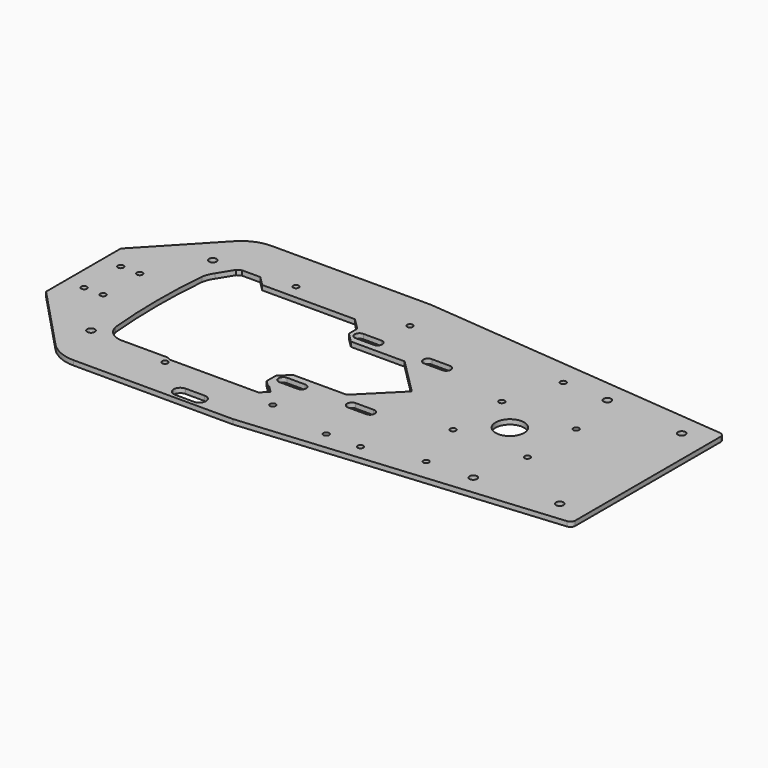
from build123d import *

# Parameters (mm, degrees)
F0_R     = 2
F0_R_2   = 1.5
F0_R_3   = 7.5
F1_DEPTH = 2.5


# Not quite as in the source:
# - ends of sketch curves that miss each other by under 0.0002 mm in the source are joined


with BuildPart() as f1:
    # F0 (on Top) → F1 (new body)
    with BuildSketch(Plane.XY):
        with BuildLine():
            Line((-115.919333, 58.73247), (-148.25, 24.5))
            Line((-148.25, 24.5), (-148.25, -24.5))
            Line((-148.25, -24.5), (-115.919333, -58.732471))
            ThreePointArc((-115.919333, -58.732471), (-109.2958427864, -63.3664016249), (-101.37907, -65))
            Line((-101.37907, -65), (-17.75, -65))
            Line((-17.75, -65), (145.974987, -50.205574))
            ThreePointArc((145.974987, -50.205574), (147.5955984677, -49.4020650272), (148.25, -47.715718))
            Line((148.25, -47.715718), (148.25, -36.5))
            Line((148.25, -36.5), (148.25, 47.715717))
            ThreePointArc((148.25, 47.715717), (147.5955984677, 49.4020640272), (145.9749869631, 50.2055725915))
            Line((145.9749869631, 50.2055725915), (-17.75, 65))
            Line((-17.75, 65), (-101.37907, 65))
            ThreePointArc((-101.37907, 65), (-109.2958431202, 63.366401481), (-115.919333, 58.73247))
        make_face()
        with Locations((-112.25, -40)):
            Circle(F0_R, mode=Mode.SUBTRACT)
        with BuildLine():
            ThreePointArc((-49.75, -63), (-52.2248737342, -61.9748737342), (-53.25, -59.5))
            ThreePointArc((-53.25, -59.5), (-52.2248737342, -57.0251262658), (-49.75, -56))
            Line((-49.75, -56), (-39.75, -56))
            ThreePointArc((-39.75, -56), (-37.2751262658, -57.0251262658), (-36.25, -59.5))
            ThreePointArc((-36.25, -59.5), (-37.2751262658, -61.9748737342), (-39.75, -63))
            Line((-39.75, -63), (-49.75, -63))
        make_face(mode=Mode.SUBTRACT)
        with Locations((-71, -43)):
            Circle(F0_R_2, mode=Mode.SUBTRACT)
        with Locations((-12.75, -45)):
            Circle(F0_R_2, mode=Mode.SUBTRACT)
        with Locations((-138.25, -12)):
            Circle(F0_R_2, mode=Mode.SUBTRACT)
        with Locations((-128.25, -12)):
            Circle(F0_R_2, mode=Mode.SUBTRACT)
        with BuildLine():
            ThreePointArc((-23.25, -27.5), (-25.017766953, -26.767766953), (-25.75, -25))
            ThreePointArc((-25.75, -25), (-25.017766953, -23.232233047), (-23.25, -22.5))
            Line((-23.25, -22.5), (-13.75, -22.5))
            ThreePointArc((-13.75, -22.5), (-11.982233047, -23.232233047), (-11.25, -25))
            ThreePointArc((-11.25, -25), (-11.982233047, -26.767766953), (-13.75, -27.5))
            Line((-13.75, -27.5), (-23.25, -27.5))
        make_face(mode=Mode.SUBTRACT)
        with Locations((20.5, -51.5)):
            Circle(F0_R_2, mode=Mode.SUBTRACT)
        with Locations((38.5, -51.5)):
            Circle(F0_R_2, mode=Mode.SUBTRACT)
        with Locations((67.75, -45)):
            Circle(F0_R_2, mode=Mode.SUBTRACT)
        with Locations((91.75, -44)):
            Circle(F0_R, mode=Mode.SUBTRACT)
        with Locations((134, -40)):
            Circle(F0_R, mode=Mode.SUBTRACT)
        with BuildLine():
            ThreePointArc((12.75, -27.5), (10.982233047, -26.767766953), (10.25, -25))
            ThreePointArc((10.25, -25), (10.982233047, -23.232233047), (12.75, -22.5))
            Line((12.75, -22.5), (22.25, -22.5))
            ThreePointArc((22.25, -22.5), (24.017766953, -23.232233047), (24.75, -25))
            ThreePointArc((24.75, -25), (24.017766953, -26.767766953), (22.25, -27.5))
            Line((22.25, -27.5), (12.75, -27.5))
        make_face(mode=Mode.SUBTRACT)
        with Locations((58.75, -16)):
            Circle(F0_R_2, mode=Mode.SUBTRACT)
        with Locations((97.75, -16)):
            Circle(F0_R_2, mode=Mode.SUBTRACT)
        with Locations((-138.25, 12)):
            Circle(F0_R_2, mode=Mode.SUBTRACT)
        with Locations((-128.25, 12)):
            Circle(F0_R_2, mode=Mode.SUBTRACT)
        with BuildLine():
            ThreePointArc((-106.6046121633, 25.7917838577), (-105.7465725985, 28.7775878211), (-104.2499995126, 31.4999996564))
            Line((-104.2499995126, 31.4999996564), (-99.481118, 39.303625))
            Line((-99.481118, 39.303625), (-97.347914, 40.5))
            Line((-97.347914, 40.5), (-87.75, 40.5))
            Line((-87.75, 40.5), (-85.25, 38))
            Line((-85.25, 38), (-82.75, 35.5))
            Line((-82.75, 35.5), (-34, 35.5))
            Line((-34, 35.5), (-28, 29.5))
            Line((-28, 29.5), (-28, 24))
            Line((-28, 24), (-23, 19))
            Line((-23, 19), (5.25, 19))
            Line((5.25, 19), (24, 0.25))
            Line((24, 0.25), (24, -0.25))
            Line((24, -0.25), (5.25, -19))
            Line((5.25, -19), (-23, -19))
            Line((-23, -19), (-28, -24))
            Line((-28, -24), (-28, -30))
            Line((-28, -30), (-25, -33))
            Line((-25, -33), (-24.25, -33))
            Line((-24.25, -33), (-20.75, -36.5))
            Line((-20.75, -36.5), (-24.25, -40))
            Line((-24.25, -40), (-70.75, -40))
            Line((-70.75, -40), (-73, -39))
            Line((-73, -39), (-96.75, -39))
            ThreePointArc((-96.75, -39), (-102.9744154707, -36.7847551324), (-106.3997748707, -31.1351909734))
            ThreePointArc((-106.3997748707, -31.1351909734), (-107.7934268918, -2.6763496917), (-106.6046121633, 25.7917838577))
        make_face(mode=Mode.SUBTRACT)
        with BuildLine():
            ThreePointArc((-23.25, 22.5), (-25.017766953, 23.232233047), (-25.75, 25))
            ThreePointArc((-25.75, 25), (-25.017766953, 26.767766953), (-23.25, 27.5))
            Line((-23.25, 27.5), (-13.75, 27.5))
            ThreePointArc((-13.75, 27.5), (-11.982233047, 26.767766953), (-11.25, 25))
            ThreePointArc((-11.25, 25), (-11.982233047, 23.232233047), (-13.75, 22.5))
            Line((-13.75, 22.5), (-23.25, 22.5))
        make_face(mode=Mode.SUBTRACT)
        with Locations((-112.25, 40)):
            Circle(F0_R, mode=Mode.SUBTRACT)
        with Locations((-71, 43)):
            Circle(F0_R_2, mode=Mode.SUBTRACT)
        with Locations((-12.75, 45)):
            Circle(F0_R_2, mode=Mode.SUBTRACT)
        with Locations((58.75, 16)):
            Circle(F0_R_2, mode=Mode.SUBTRACT)
        with BuildLine():
            ThreePointArc((12.75, 22.5), (10.982233047, 23.232233047), (10.25, 25))
            ThreePointArc((10.25, 25), (10.982233047, 26.767766953), (12.75, 27.5))
            Line((12.75, 27.5), (22.25, 27.5))
            ThreePointArc((22.25, 27.5), (24.017766953, 26.767766953), (24.75, 25))
            ThreePointArc((24.75, 25), (24.017766953, 23.232233047), (22.25, 22.5))
            Line((22.25, 22.5), (12.75, 22.5))
        make_face(mode=Mode.SUBTRACT)
        with Locations((75.75, 0)):
            Circle(F0_R_3, mode=Mode.SUBTRACT)
        with Locations((97.75, 16)):
            Circle(F0_R_2, mode=Mode.SUBTRACT)
        with Locations((67.75, 45)):
            Circle(F0_R_2, mode=Mode.SUBTRACT)
        with Locations((91.75, 44)):
            Circle(F0_R, mode=Mode.SUBTRACT)
        with Locations((134, 40)):
            Circle(F0_R, mode=Mode.SUBTRACT)
    extrude(amount=F1_DEPTH)


solid = f1.part
